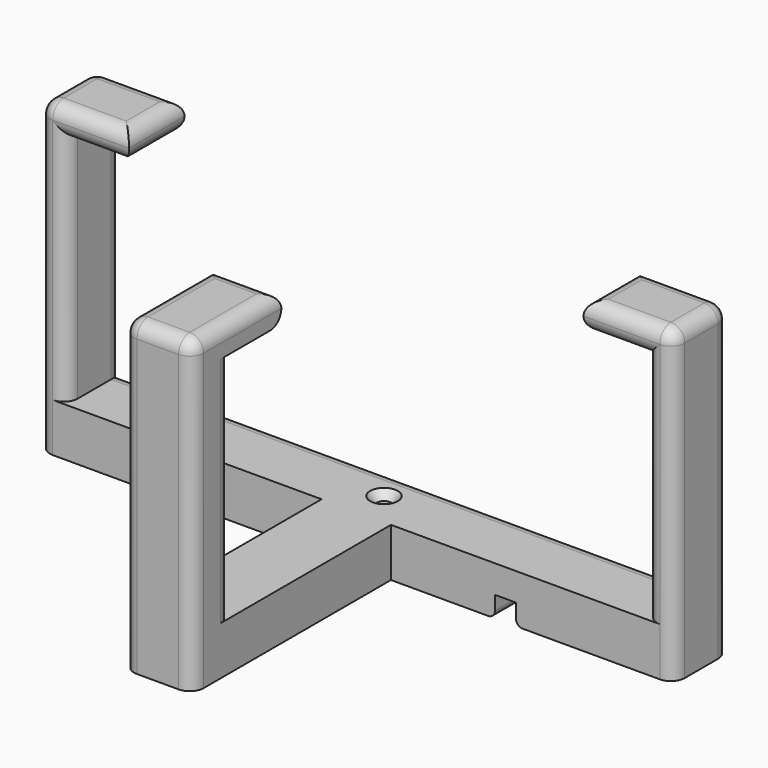
from build123d import *

# Parameters (mm, degrees)
F0_W            = 91.5
F0_H            = 7
F1_DEPTH        = 5
F2_W            = 5
F2_H            = 40.75
F3_DEPTH        = 3.5
F4_W            = 4
F4_H            = 10
F5_DEPTH        = 37.5
F6_W            = 4
F6_H            = 10
F7_DEPTH        = 37.5
F8_W            = 10
F8_H            = 7
F9_DEPTH        = 37.5
F10_W           = 10
F10_H           = 4
F11_DEPTH       = 9
F12_W           = 10
F12_H           = 4
F13_DEPTH       = 9
F14_W           = 10
F14_H           = 4
F15_DEPTH       = 9
F16_R           = 1.99999
F18_D           = 2
F18_DEPTH       = 18
F18_CSINK_D     = 4
F18_CSINK_ANGLE = 82
F18_TIP         = 0.600860619
F19_W           = 3
F19_H           = 10
F20_DEPTH       = 3
F21_R           = 1
F22_W           = 5
F22_H           = 27.7060836997
F23_DEPTH       = 0.5


# Not quite as in the source:
# - a fillet or chamfer is up to 0.001 mm smaller than in the source, because OpenCascade refuses the exact size


with BuildPart() as f1:
    # F0 (on Front) → F1 (new body, symmetric)
    with BuildSketch(Plane.XZ):
        Rectangle(F0_W, F0_H)
    extrude(amount=F1_DEPTH, both=True)

    # F2 (on Top) → F3 (join, symmetric)
    with BuildSketch(Plane.XY):
        with Locations((-2.5, -20.375)):
            Rectangle(F2_W, F2_H)
        with Locations((2.5, -20.375)):
            Rectangle(F2_W, F2_H)
    extrude(amount=F3_DEPTH, both=True)

    # F4 (on face) → F5 (join)
    with BuildSketch(Plane.XY.offset(3.5)):
        with Locations((-43.75, 0)):
            Rectangle(F4_W, F4_H)
    extrude(amount=F5_DEPTH)

    # F6 (on face) → F7 (join)
    with BuildSketch(Plane.XY.offset(3.5)):
        with Locations((43.75, 0)):
            Rectangle(F6_W, F6_H)
    extrude(amount=F7_DEPTH)

    # F8 (on face) → F9 (join)
    with BuildSketch(Plane.XY.offset(3.5)):
        with Locations((0, -37.25)):
            Rectangle(F8_W, F8_H)
    extrude(amount=F9_DEPTH)

    # F10 (on face) → F11 (join)
    with BuildSketch(Plane(origin=(0, -33.75, 0), x_dir=(-1, 0, 0), z_dir=(0, 1, 0))):
        with Locations((0, 39)):
            Rectangle(F10_W, F10_H)
    extrude(amount=F11_DEPTH)

    # F12 (on face) → F13 (join)
    with BuildSketch(Plane(origin=(41.75, 0, 0), x_dir=(0, -1, 0), z_dir=(-1, 0, 0))):
        with Locations((0, 39)):
            Rectangle(F12_W, F12_H)
    extrude(amount=F13_DEPTH)

    # F14 (on face) → F15 (join)
    with BuildSketch(Plane.YZ.offset(-41.75)):
        with Locations((0, 39)):
            Rectangle(F14_W, F14_H)
    extrude(amount=F15_DEPTH)

    # F16 (radius 2 in the source; OpenCascade refuses exactly that, so slightly less here)
    f16_edges = [f1.edges().sort_by_distance(p)[0] for p in [
        (0, 5, 3.5),
        (41.75, 5, 20.25),
        (37.25, 5, 37),
        (-41.75, 5, 20.25),
        (-37.25, 5, 37),
        (32.75, 0, 41),
        (39.25, 5, 41),
        (45.75, 5, 18.75),
        (-45.75, 5, 18.75),
        (-39.25, 5, 41),
        (-32.75, 0, 41),
        (0, -24.75, 41),
        (-5, -33.75, 20.25),
        (5, -33.75, 20.25),
        (-41.75, -5, 20.25),
        (41.75, -5, 20.25),
        (-37.25, -5, 37),
        (37.25, -5, 37),
        (-45.75, 0, 41),
        (45.75, 0, 41),
        (0, -40.75, 41),
        (5, -32.75, 41),
        (-5, -32.75, 41),
        (0, -24.75, 37),
        (-5, -40.75, 18.75),
        (5, -40.75, 18.75),
        (39.25, -5, 41),
        (-39.25, -5, 41),
        (-45.75, -5, 18.75),
        (45.75, -5, 18.75),
        (-32.75, 0, 37),
        (32.75, 0, 37),
    ]]
    fillet(f16_edges, radius=F16_R)

    # F18
    with Locations(Plane.XY.offset(3.5)):
        with Locations((0, 0)):
            CounterSinkHole(F18_D / 2, F18_CSINK_D / 2, depth=F18_DEPTH, counter_sink_angle=F18_CSINK_ANGLE)
            with Locations((0, 0, -(F18_DEPTH + F18_TIP / 2))):  # 118° drill point
                Cone(0, F18_D / 2, F18_TIP, mode=Mode.SUBTRACT)

    # F19 (on face) → F20 (cut)
    with BuildSketch(Plane(origin=(0, 0, -3.5), x_dir=(1, 0, 0), z_dir=(0, 0, -1))):
        with Locations((21.5, 0)):
            Rectangle(F19_W, F19_H)
        with Locations((-22.5, 0)):
            Rectangle(F19_W, F19_H)
    extrude(amount=-F20_DEPTH, mode=Mode.SUBTRACT)

    # F21
    f21_edges = [f1.edges().sort_by_distance(p)[0] for p in [
        (20, 0, -3.5),
        (23, 0, -3.5),
        (-21, 0, -3.5),
        (-24, 0, -3.5),
    ]]
    fillet(f21_edges, radius=F21_R)

    # F22 (on face) → F23 (cut)
    with BuildSketch(Plane(origin=(0, 0, -3.5), x_dir=(1, 0, 0), z_dir=(0, 0, -1))):
        with Locations((0, 18.8530418498)):
            Rectangle(F22_W, F22_H)
    extrude(amount=-F23_DEPTH, mode=Mode.SUBTRACT)


solid = f1.part
